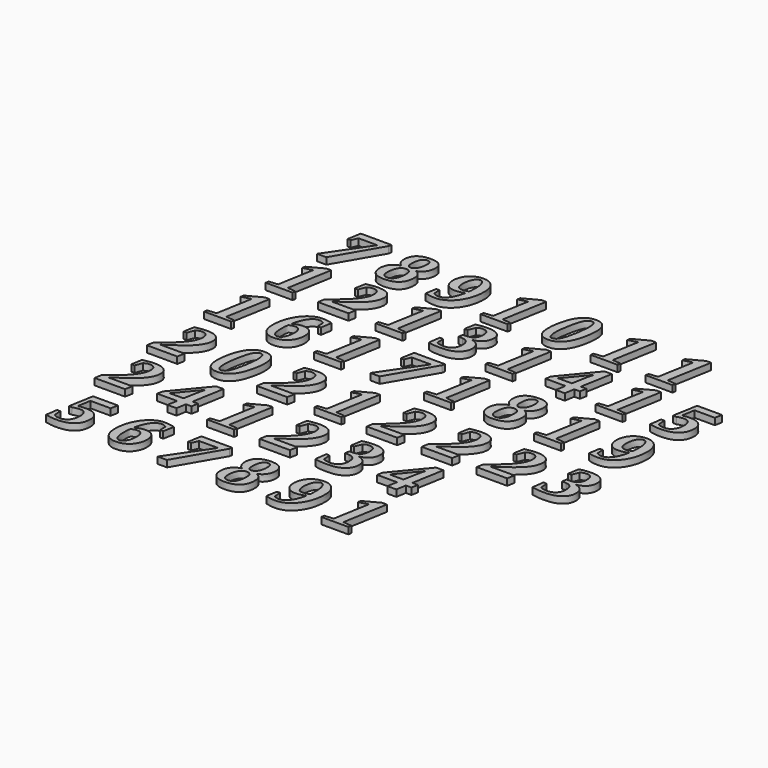
from build123d import *

# Parameters (mm, degrees)
F0_TEXT_SIZE = 22.2222222222
F1_DEPTH     = 2


# Not quite as in the source:
# - Text() gives the source's letters only with a copy of the font that has no kerning and outlines rounded to 1/6400 em; it was checked with that copy


with BuildPart() as f1:
    # F0 (on Top) → F1 (new body)
    with BuildSketch(Plane.XY):
        with Locations((-63.8358518481, 49.5567124486)):
            Text('7 8 9 1 0 1 1', F0_TEXT_SIZE, font='Tinos', font_style=FontStyle.BOLDITALIC, text_align=(TextAlign.LEFT, TextAlign.BOTTOM))
        with Locations((-63.6719614267, 30.3813766837)):
            Text('1 2 1 3 1 4 1 5', F0_TEXT_SIZE, font='Tinos', font_style=FontStyle.BOLDITALIC, text_align=(TextAlign.LEFT, TextAlign.BOTTOM))
        with Locations((-65.802551806, 9.7310103625)):
            Text('1 6 1 7 1 8 1 9', F0_TEXT_SIZE, font='Tinos', font_style=FontStyle.BOLDITALIC, text_align=(TextAlign.LEFT, TextAlign.BOTTOM))
        with Locations((-64.819201827, -12.2304888759)):
            Text('2 0 2 1 2 2 2 3', F0_TEXT_SIZE, font='Tinos', font_style=FontStyle.BOLDITALIC, text_align=(TextAlign.LEFT, TextAlign.BOTTOM))
        with Locations((-63.9997422695, -33.0447453856)):
            Text('2 4 1 2 3 4', F0_TEXT_SIZE, font='Tinos', font_style=FontStyle.BOLDITALIC, text_align=(TextAlign.LEFT, TextAlign.BOTTOM))
        with Locations((-61.7052540183, -55.1701385379)):
            Text('5 6 7 8 9 1', F0_TEXT_SIZE, font='Tinos', font_style=FontStyle.BOLDITALIC, text_align=(TextAlign.LEFT, TextAlign.BOTTOM))
    extrude(amount=F1_DEPTH)


solid = f1.part
